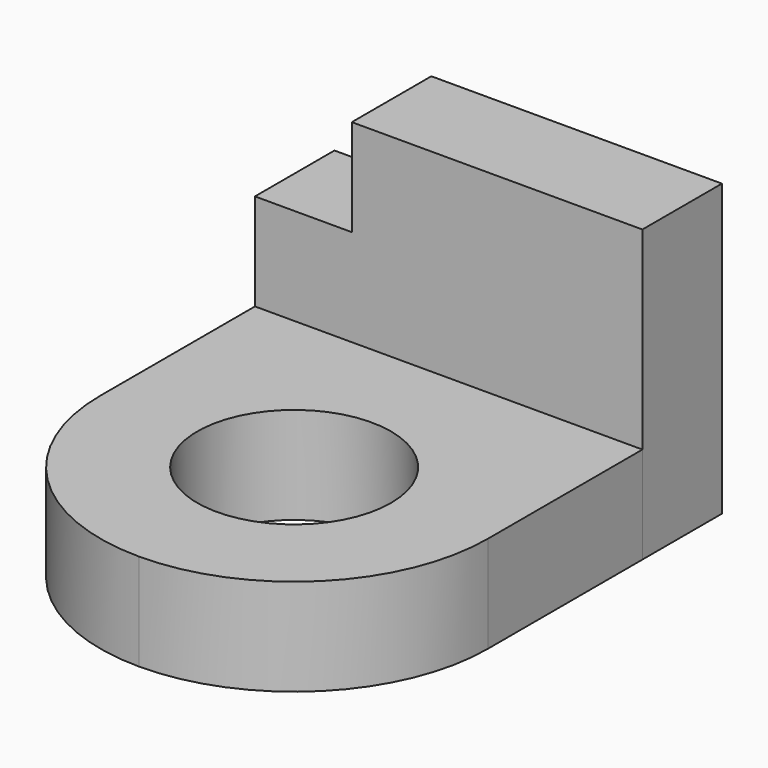
from build123d import *

# Parameters (mm, degrees)
F0_W     = 50.8
F0_H     = 63.754
F1_DEPTH = 12.7
F2_W     = 50.8
F2_H     = 13.0302
F3_DEPTH = 38.1
F4_W     = 12.7
F4_H     = 13.0302
F5_DEPTH = 12.7
F6_R     = 25.39999
F7_R     = 12.7
F8_DEPTH = 12.701


# Not quite as in the source:
# - a fillet or chamfer is up to 0.001 mm smaller than in the source, because OpenCascade refuses the exact size


with BuildPart() as f1:
    # F0 (on Top) → F1 (new body)
    with BuildSketch(Plane.XY):
        Rectangle(F0_W, F0_H)
    extrude(amount=F1_DEPTH)

    # F2 (on Top) → F3 (join)
    with BuildSketch(Plane.XY):
        with Locations((1.8626e-06, 25.3619)):
            Rectangle(F2_W, F2_H)
    extrude(amount=F3_DEPTH)

    # F4 (on face) → F5 (cut)
    with BuildSketch(Plane.XY.offset(38.1)):
        with Locations((-19.0499981374, 25.3619)):
            Rectangle(F4_W, F4_H)
    extrude(amount=-F5_DEPTH, mode=Mode.SUBTRACT)

    # F6 (radius 25.4 in the source; OpenCascade refuses exactly that, so slightly less here)
    f6_edges = [f1.edges().sort_by_distance(p)[0] for p in [
        (-25.4, -31.877, 6.35),
        (25.4, -31.877, 6.35),
    ]]
    fillet(f6_edges, radius=F6_R)

    # F7 (on face) → F8 (cut, through all)
    with BuildSketch(Plane.XY.offset(12.7)):
        with Locations((0, -6.477)):
            Circle(F7_R)
    extrude(amount=-F8_DEPTH, mode=Mode.SUBTRACT)


solid = f1.part
